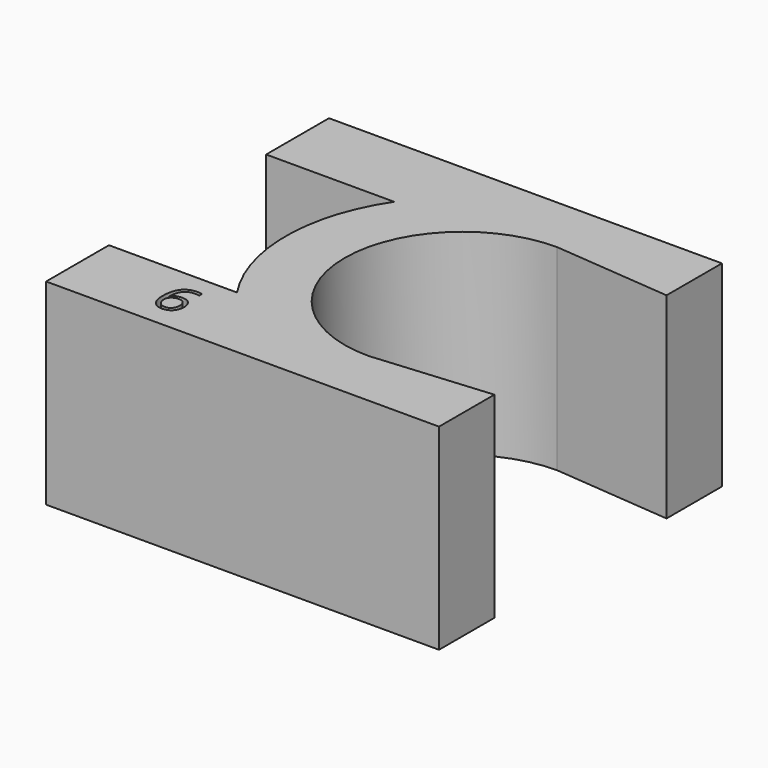
from build123d import *

# Parameters (mm, degrees)
F1_DEPTH     = 5
F2_TEXT_SIZE = 1.367309273
F3_DEPTH     = 2


# Not quite as in the source:
# - Text() gives the source's letters only with a copy of the font that has no kerning and outlines rounded to 1/6400 em; it was checked with that copy


with BuildPart() as f1:
    # F0 (on Top) → F1 (new body)
    with BuildSketch(Plane.XY):
        with BuildLine():
            ThreePointArc((0, -3), (-3, 0), (0, 3))
            Line((0, 3), (3, 2.7375340094))
            Line((3, 2.7375340094), (3, 4.5))
            Line((3, 4.5), (0, 4.5))
            Line((0, 4.5), (-7, 4.5))
            Line((-7, 4.5), (-7, 2.5))
            Line((-7, 2.5), (-3.7416573868, 2.5))
            ThreePointArc((-3.7416573868, 2.5), (-4.5, 0), (-3.7416573868, -2.5))
            Line((-3.7416573868, -2.5), (-7, -2.5))
            Line((-7, -2.5), (-7, -4.5))
            Line((-7, -4.5), (0, -4.5))
            Line((0, -4.5), (3, -4.5))
            Line((3, -4.5), (3, -2.7375340094))
            Line((3, -2.7375340094), (0, -3))
        make_face()
    extrude(amount=F1_DEPTH)

    # F2 (on face) → F3 (cut)
    with BuildSketch(Plane.XY.offset(5)):
        with Locations((-4.8830686137, -3.9612893015)):
            Text('6', F2_TEXT_SIZE, font='Open Sans', text_align=(TextAlign.LEFT, TextAlign.BOTTOM))
    extrude(amount=-F3_DEPTH, mode=Mode.SUBTRACT)


solid = f1.part
